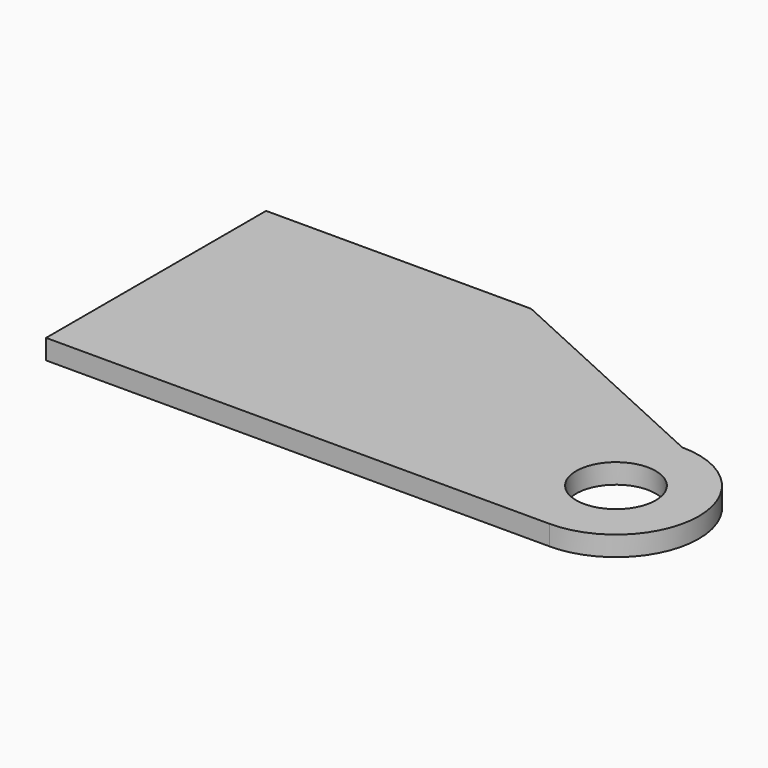
from build123d import *

# Parameters (mm, degrees)
F0_R     = 6
F1_DEPTH = 3


# Not quite as in the source:
# - a feature names something its author has since deleted; it is built from what else it names


with BuildPart() as f1:
    # F0 (on Top) → F1 (new body)
    with BuildSketch(Plane.XY):
        with BuildLine():
            Line((-36, 29), (-76, 29))
            Line((-76, 29), (-76, -12.5))
            Line((-76, -12.5), (0, -12.5))
            ThreePointArc((0, -12.5), (12.5, 0), (0, 12.5))
            Line((0, 12.5), (-36, 29))
        make_face()
        Circle(F0_R, mode=Mode.SUBTRACT)
    extrude(amount=-F1_DEPTH)


solid = f1.part
